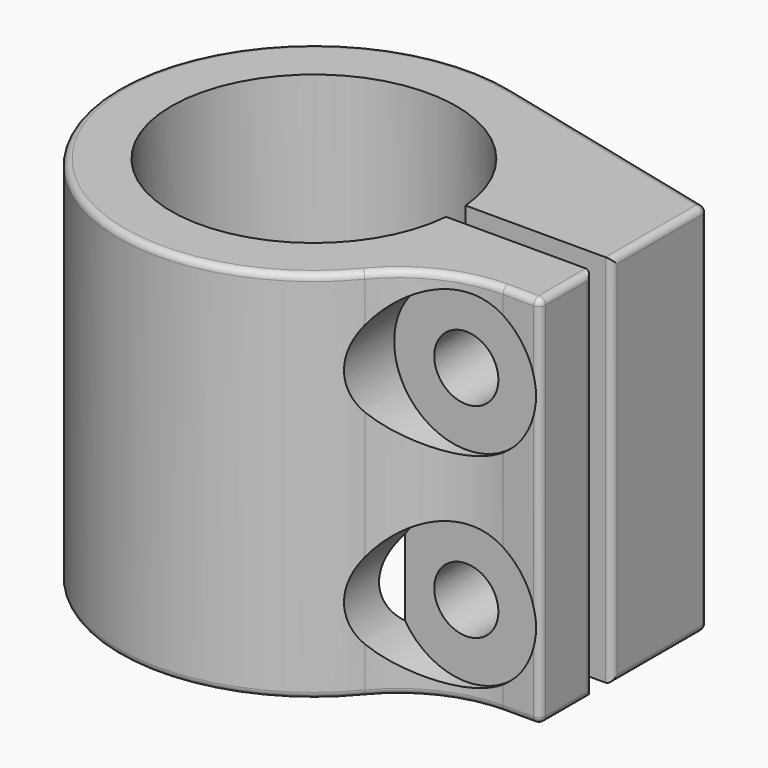
from build123d import *

# Parameters (mm, degrees)
F1_DEPTH       = 14.605
F2_DEPTH       = 14.605
F5_D           = 5
F5_DEPTH       = 25.4
F5_START       = 7.9375001
F5_CBORE_D     = 11.25
F5_CBORE_DEPTH = 0.254
F5_TIP         = 1.5021515476
F6_T1_DEPTH    = 10.0794155694
F6_T3_DEPTH    = 28.194
F6_T5_DEPTH    = 18.9996845391
F6_T7_DEPTH    = 2.4015609751
F6_T9_DEPTH    = 5.842
F6_T11_DEPTH   = 31.75
F6_T16_DEPTH   = 0.508
F6_T22_DEPTH   = 0.508
F6_S27_W       = 0.508
F6_S27_H       = 0.508
F6_T28_DEPTH   = 0.508
F6_S33_W       = 0.508
F6_S33_H       = 0.508
F6_T34_DEPTH   = 0.508
F6_T38_ANGLE   = 244.2276643477
F6_T40_ANGLE   = 244.2276643477
F6_T42_ANGLE   = 50.3943476061
F6_T44_ANGLE   = 50.3943476061


# Not quite as in the source:
# - a fillet or chamfer that OpenCascade refuses, or shapes differently, is made with other operations: its cross-section is extruded or revolved along the edge and cut away or added
# - two fillets or chamfers of one size are made in one step
# - a feature names something its author has since deleted; it is built from what else it names


with BuildPart() as f1:
    # F0 (on Top) → F1 (new body, symmetric)
    with BuildSketch(Plane.XY):
        with BuildLine():
            ThreePointArc((13.0462755126, -0.9525), (-13.081, 0), (13.0462755126, 0.9525))
            Line((13.0462755126, 0.9525), (22.479, 0.9525))
            Line((22.479, 0.9525), (22.479, 10.16))
            Line((22.479, 10.16), (3.6438553339, 14.7979700738))
            ThreePointArc((3.6438553339, 14.7979700738), (-14.4708707602, -4.7803241985), (11.741663415, -9.7155))
            ThreePointArc((11.741663415, -9.7155), (15.243974888, -6.999243776), (19.5694390249, -6.0325))
            Line((19.5694390249, -6.0325), (22.479, -6.0325))
            Line((22.479, -6.0325), (22.479, -0.9525))
            Line((22.479, -0.9525), (13.0462755126, -0.9525))
        make_face()
    extrude(amount=F1_DEPTH, both=True)

    # F0 (on Top) → F2 (join, through all)
    with BuildSketch(Plane.XY):
        with BuildLine():
            Line((11.0716033166, 0.9525), (13.0462755126, 0.9525))
            ThreePointArc((13.0462755126, 0.9525), (-13.081, 0), (13.0462755126, -0.9525))
            Line((13.0462755126, -0.9525), (11.0716033166, -0.9525))
            ThreePointArc((11.0716033166, -0.9525), (-11.1125, 0), (11.0716033166, 0.9525))
        make_face()
    extrude(amount=F2_DEPTH)

    # F5
    # its depths count from where the whole tool has entered the part; down to there all is cleared
    with Locations(Plane.XZ.offset(13.97).offset(-F5_START)):
        with Locations((16.51, 7.9626224567), (16.51, -7.9626224567)):
            CounterBoreHole(F5_D / 2, F5_CBORE_D / 2, F5_CBORE_DEPTH, depth=F5_DEPTH)
            with Locations((0, 0, -(F5_DEPTH + F5_TIP / 2))):  # 118° drill point
                Cone(0, F5_D / 2, F5_TIP, mode=Mode.SUBTRACT)

    # F6: fillet of radius 0.508 on 16 edges, made by hand

    # F6_s2 → F6_t1 (cut)
    with BuildSketch(Plane.XZ.offset(-9.7619155694)):
        with BuildLine():
            ThreePointArc((21.971, -14.605), (22.3302102448, -14.4562102448), (22.479, -14.097))
            Line((22.479, -14.097), (22.479, -14.605))
            Line((22.479, -14.605), (21.971, -14.605))
        make_face()
        with BuildLine():
            ThreePointArc((21.971, 14.605), (22.3302102448, 14.4562102448), (22.479, 14.097))
            Line((22.479, 14.097), (22.479, 14.605))
            Line((22.479, 14.605), (21.971, 14.605))
        make_face()
    extrude(amount=F6_T1_DEPTH, mode=Mode.SUBTRACT)

    # F6_s4 → F6_t3 (cut)
    with BuildSketch(Plane.XY.offset(-14.097)):
        with BuildLine():
            ThreePointArc((22.0924618445, 10.2551812386), (22.370854109, 10.0752535523), (22.479, 9.7619155694))
            Line((22.479, 9.7619155694), (22.479, 10.16))
            Line((22.479, 10.16), (22.0924618445, 10.2551812386))
        make_face()
        with BuildLine():
            ThreePointArc((21.971, -6.0325), (22.3302102448, -5.8837102448), (22.479, -5.5245))
            Line((22.479, -5.5245), (22.479, -6.0325))
            Line((22.479, -6.0325), (21.971, -6.0325))
        make_face()
    extrude(amount=F6_T3_DEPTH, mode=Mode.SUBTRACT)

    # F6_s6 → F6_t5 (cut)
    with BuildSketch(Plane(origin=(18.4486065106, -4.5427888353, 0), x_dir=(0, 0, 1), z_dir=(-0.9709954117, 0.239098119, 0))):
        with BuildLine():
            ThreePointArc((14.097, 15.24), (14.4562102448, 15.0912102448), (14.605, 14.732))
            Line((14.605, 14.732), (14.605, 15.24))
            Line((14.605, 15.24), (14.097, 15.24))
        make_face()
        with BuildLine():
            ThreePointArc((-14.605, 14.732), (-14.4562102448, 15.0912102448), (-14.097, 15.24))
            Line((-14.097, 15.24), (-14.605, 15.24))
            Line((-14.605, 15.24), (-14.605, 14.732))
        make_face()
    extrude(amount=F6_T5_DEPTH, mode=Mode.SUBTRACT)

    # F6_s8 → F6_t7 (cut)
    with BuildSketch(Plane.YZ.offset(19.5694390249)):
        with BuildLine():
            ThreePointArc((-6.0325, 14.097), (-5.8837102448, 14.4562102448), (-5.5245, 14.605))
            Line((-5.5245, 14.605), (-6.0325, 14.605))
            Line((-6.0325, 14.605), (-6.0325, 14.097))
        make_face()
        with BuildLine():
            ThreePointArc((-6.0325, -14.097), (-5.8837102448, -14.4562102448), (-5.5245, -14.605))
            Line((-5.5245, -14.605), (-6.0325, -14.605))
            Line((-6.0325, -14.605), (-6.0325, -14.097))
        make_face()
    extrude(amount=F6_T7_DEPTH, mode=Mode.SUBTRACT)

    # F6_s10 → F6_t9 (cut)
    with BuildSketch(Plane.XZ.offset(-0.3175)):
        with BuildLine():
            ThreePointArc((21.971, -14.605), (22.3302102448, -14.4562102448), (22.479, -14.097))
            Line((22.479, -14.097), (22.479, -14.605))
            Line((22.479, -14.605), (21.971, -14.605))
        make_face()
        with BuildLine():
            ThreePointArc((21.971, 14.605), (22.3302102448, 14.4562102448), (22.479, 14.097))
            Line((22.479, 14.097), (22.479, 14.605))
            Line((22.479, 14.605), (21.971, 14.605))
        make_face()
    extrude(amount=F6_T9_DEPTH, mode=Mode.SUBTRACT)

    # F6_s12 → F6_t11 (cut)
    with BuildSketch(Plane.XY.offset(-15.875)):
        with BuildLine():
            ThreePointArc((22.479, -1.4605), (22.3302102448, -1.1012897552), (21.971, -0.9525))
            Line((21.971, -0.9525), (22.479, -0.9525))
            Line((22.479, -0.9525), (22.479, -1.4605))
        make_face()
        with BuildLine():
            ThreePointArc((21.971, 0.9525), (22.3302102448, 1.1012897552), (22.479, 1.4605))
            Line((22.479, 1.4605), (22.479, 0.9525))
            Line((22.479, 0.9525), (21.971, 0.9525))
        make_face()
    extrude(amount=F6_T11_DEPTH, mode=Mode.SUBTRACT)


with BuildPart() as f6_tool14:
    # F6_s15 → F6_t16 (new body)
    with BuildSketch(Plane.XY.offset(-14.097)):
        Polygon((21.971, 9.7619155694), (22.0924618445, 10.2551812386), (22.479, 10.16), (22.479, 9.7619155694), align=None)
    extrude(amount=-F6_T16_DEPTH)

    # F6_s17 → F6_t18 (revolve, cut)
    with BuildSketch(Plane(origin=(21.971, 9.7619155694, -14.097), x_dir=(-0.7871143878, -0.6168070529, 0), z_dir=(0.6168070529, -0.7871143878, 0))):
        with BuildLine():
            ThreePointArc((0, -0.508), (0.508, 0), (0, 0.508))
            Line((0, 0.508), (0, -0.508))
        make_face()
    revolve(axis=Axis((21.971, 9.7619155694, -14.097), (0, 0, -1)), mode=Mode.SUBTRACT)


with BuildPart() as f1_1:
    add(f1.part)

    # F6_t13: cut F6_tool14
    add(f6_tool14.part, mode=Mode.SUBTRACT)


with BuildPart() as f6_tool20:
    # F6_s21 → F6_t22 (new body)
    with BuildSketch(Plane.XY.offset(14.097)):
        Polygon((21.971, 9.7619155694), (22.479, 9.7619155694), (22.479, 10.16), (22.0924618445, 10.2551812386), align=None)
    extrude(amount=F6_T22_DEPTH)

    # F6_s23 → F6_t24 (revolve, cut)
    with BuildSketch(Plane(origin=(21.971, 9.7619155694, 14.097), x_dir=(-0.7871143878, -0.6168070529, 0), z_dir=(-0.6168070529, 0.7871143878, 0))):
        with BuildLine():
            ThreePointArc((0, -0.508), (0.508, 0), (0, 0.508))
            Line((0, 0.508), (0, -0.508))
        make_face()
    revolve(axis=Axis((21.971, 9.7619155694, 14.097), (0, 0, 1)), mode=Mode.SUBTRACT)


with BuildPart() as f1_2:
    add(f1_1.part)

    # F6_t19: cut F6_tool20
    add(f6_tool20.part, mode=Mode.SUBTRACT)


with BuildPart() as f6_tool26:
    # F6_s27 → F6_t28 (new body)
    with BuildSketch(Plane.XZ.offset(5.5245)):
        with Locations((22.225, 14.351)):
            Rectangle(F6_S27_W, F6_S27_H)
    extrude(amount=F6_T28_DEPTH)

    # F6_s29 → F6_t30 (revolve, cut)
    with BuildSketch(Plane(origin=(21.971, -5.5245, 14.097), x_dir=(-0.7071067812, 0, -0.7071067812), z_dir=(-0.7071067812, 0, 0.7071067812))):
        with BuildLine():
            ThreePointArc((0, -0.508), (0.508, 0), (0, 0.508))
            Line((0, 0.508), (0, -0.508))
        make_face()
    revolve(axis=Axis((21.971, -5.5245, 14.097), (0, -1, 0)), mode=Mode.SUBTRACT)


with BuildPart() as f1_3:
    add(f1_2.part)

    # F6_t25: cut F6_tool26
    add(f6_tool26.part, mode=Mode.SUBTRACT)


with BuildPart() as f6_tool32:
    # F6_s33 → F6_t34 (new body)
    with BuildSketch(Plane.XZ.offset(5.5245)):
        with Locations((22.225, -14.351)):
            Rectangle(F6_S33_W, F6_S33_H)
    extrude(amount=F6_T34_DEPTH)

    # F6_s35 → F6_t36 (revolve, cut)
    with BuildSketch(Plane(origin=(21.971, -5.5245, -14.097), x_dir=(-0.7071067812, 0, 0.7071067812), z_dir=(0.7071067812, 0, 0.7071067812))):
        with BuildLine():
            ThreePointArc((0, -0.508), (0.508, 0), (0, 0.508))
            Line((0, 0.508), (0, -0.508))
        make_face()
    revolve(axis=Axis((21.971, -5.5245, -14.097), (0, -1, 0)), mode=Mode.SUBTRACT)


with BuildPart() as f1_4:
    add(f1_3.part)

    # F6_t31: cut F6_tool32
    add(f6_tool32.part, mode=Mode.SUBTRACT)

    # F6_s37 → F6_t38 (revolve, cut)
    with BuildSketch(Plane(origin=(0, 0, 0), x_dir=(0, 0, 1), z_dir=(0.9709954117, -0.239098119, 0))):
        with BuildLine():
            ThreePointArc((-14.097, -15.24), (-14.4562102448, -15.0912102448), (-14.605, -14.732))
            Line((-14.605, -14.732), (-14.605, -15.24))
            Line((-14.605, -15.24), (-14.097, -15.24))
        make_face()
    revolve(axis=Axis((0, 0, -14.605), (0, 0, 1)), revolution_arc=F6_T38_ANGLE, mode=Mode.SUBTRACT)

    # F6_s39 → F6_t40 (revolve, cut)
    with BuildSketch(Plane(origin=(0, 0, 0), x_dir=(0, 0, 1), z_dir=(0.9709954117, -0.239098119, 0))):
        with BuildLine():
            ThreePointArc((14.097, -15.24), (14.4562102448, -15.0912102448), (14.605, -14.732))
            Line((14.605, -14.732), (14.605, -15.24))
            Line((14.605, -15.24), (14.097, -15.24))
        make_face()
    revolve(axis=Axis((0, 0, 14.605), (0, 0, 1)), revolution_arc=F6_T40_ANGLE, mode=Mode.SUBTRACT)

    # F6_s41 → F6_t42 (revolve, cut)
    with BuildSketch(Plane(origin=(0, 0, 0), x_dir=(0, 0, 1), z_dir=(-0.6375, -0.7704503553, 0))):
        with BuildLine():
            ThreePointArc((-14.097, -15.24), (-14.4562102448, -15.0912102448), (-14.605, -14.732))
            Line((-14.605, -14.732), (-14.605, -15.24))
            Line((-14.605, -15.24), (-14.097, -15.24))
        make_face()
    revolve(axis=Axis((19.5694390249, -16.1925, -14.605), (0, 0, -1)), revolution_arc=F6_T42_ANGLE, mode=Mode.SUBTRACT)

    # F6_s43 → F6_t44 (revolve, cut)
    with BuildSketch(Plane(origin=(0, 0, 0), x_dir=(0, 0, 1), z_dir=(-0.6375, -0.7704503553, 0))):
        with BuildLine():
            ThreePointArc((14.605, -14.732), (14.4562102448, -15.0912102448), (14.097, -15.24))
            Line((14.097, -15.24), (14.605, -15.24))
            Line((14.605, -15.24), (14.605, -14.732))
        make_face()
    revolve(axis=Axis((19.5694390249, -16.1925, 14.605), (0, 0, -1)), revolution_arc=F6_T44_ANGLE, mode=Mode.SUBTRACT)


solid = f1_4.part
